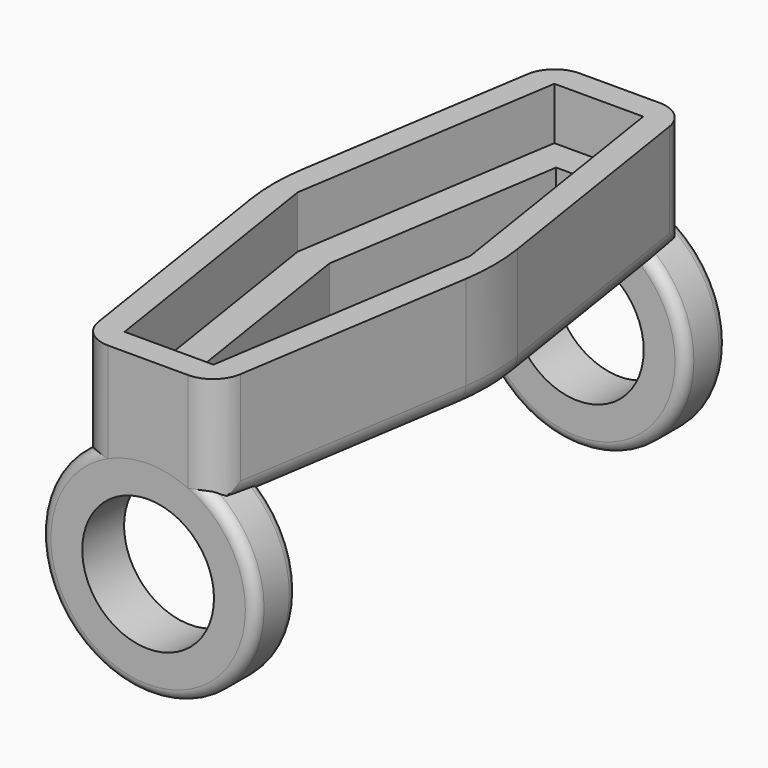
from build123d import *

# Parameters (mm, degrees)
F1_DEPTH     = 6
F2_DEPTH     = 11
F3_R         = 10.3
F4_DEPTH     = 5
F8_R         = 2
F9_R         = 1
F9_2_R       = 1
F10_T1_DEPTH = 21.8452325787
F11_T1_DEPTH = 18.7849894416
F11_T4_ANGLE = 17.6997661969
F11_T6_ANGLE = 17.6997661969


# Not quite as in the source:
# - a fillet or chamfer that OpenCascade refuses, or shapes differently, is made with other operations: its cross-section is extruded or revolved along the edge and cut away or added


with BuildPart() as f1:
    # F0 (on Top) → F1 (new body)
    with BuildSketch(Plane.XY):
        Polygon((4.25, -25.6904651573), (8.25, 0), (4.25, 25.6904651573), (0, 25.6904651573), (-4.25, 25.6904651573), (-8.25, 0), (-4.25, -25.6904651573), (0, -25.6904651573), align=None)
        Polygon((0, 22.6904651573), (1.6809534843, 22.6904651573), (5.2138541178, 0), (1.6809534843, -22.6904651573), (0, -22.6904651573), (-1.6809534843, -22.6904651573), (-5.2138541178, 0), (-1.6809534843, 22.6904651573), align=None, mode=Mode.SUBTRACT)
    extrude(amount=F1_DEPTH)

    # F0 (on Top) → F2 (join)
    with BuildSketch(Plane.XY):
        Polygon((-6.3908720964, 28.1904651573), (-10.7801215685, 0), (-6.3908720964, -28.1904651573), (0, -28.1904651573), (6.3908720964, -28.1904651573), (10.7801215685, 0), (6.3908720964, 28.1904651573), (0, 28.1904651573), align=None)
        Polygon((4.25, 25.6904651573), (8.25, 0), (4.25, -25.6904651573), (0, -25.6904651573), (-4.25, -25.6904651573), (-8.25, 0), (-4.25, 25.6904651573), (0, 25.6904651573), align=None, mode=Mode.SUBTRACT)
    extrude(amount=F2_DEPTH)

    # F8
    f8_edges = [f1.edges().sort_by_distance(p)[0] for p in [
        (-8.585497, -14.095233, 0),
        (-8.585497, 14.095233, 0),
        (8.585497, 14.095233, 0),
        (8.585497, -14.095233, 0),
    ]]
    fillet(f8_edges, radius=F8_R)

    # F10: fillet of radius 3 on 4 edges, made by hand

    # F10_s2 → F10_t1 (cut)
    with BuildSketch(Plane.XY.offset(-4.4226162893)):
        with BuildLine():
            ThreePointArc((-3.8218255807, -28.1904651573), (-5.7731564875, -27.4691287333), (-6.7861100219, -25.6520036189))
            Line((-6.7861100219, -25.6520036189), (-6.3908720964, -28.1904651573))
            Line((-6.3908720964, -28.1904651573), (-3.8218255807, -28.1904651573))
        make_face()
        with BuildLine():
            ThreePointArc((3.8218255807, -28.1904651573), (5.7731564875, -27.4691287333), (6.7861100219, -25.6520036189))
            Line((6.7861100219, -25.6520036189), (6.3908720964, -28.1904651573))
            Line((6.3908720964, -28.1904651573), (3.8218255807, -28.1904651573))
        make_face()
        with BuildLine():
            ThreePointArc((-3.8218255807, 28.1904651573), (-5.7731564875, 27.4691287333), (-6.7861100219, 25.6520036189))
            Line((-6.7861100219, 25.6520036189), (-6.3908720964, 28.1904651573))
            Line((-6.3908720964, 28.1904651573), (-3.8218255807, 28.1904651573))
        make_face()
        with BuildLine():
            ThreePointArc((3.8218255807, 28.1904651573), (5.7731564875, 27.4691287333), (6.7861100219, 25.6520036189))
            Line((6.7861100219, 25.6520036189), (6.3908720964, 28.1904651573))
            Line((6.3908720964, 28.1904651573), (3.8218255807, 28.1904651573))
        make_face()
    extrude(amount=F10_T1_DEPTH, mode=Mode.SUBTRACT)

    # F11: fillet of radius 20 on 2 edges, made by hand

    # F11_s2 → F11_t1 (cut)
    with BuildSketch(Plane.XY):
        with BuildLine():
            ThreePointArc((-10.3010452952, -3.0769230769), (-10.5391490203, 0), (-10.3010452952, 3.0769230769))
            Line((-10.3010452952, 3.0769230769), (-10.7801215685, 0))
            Line((-10.7801215685, 0), (-10.3010452952, -3.0769230769))
        make_face()
        with BuildLine():
            ThreePointArc((10.3010452952, 3.0769230769), (10.5391490203, 0), (10.3010452952, -3.0769230769))
            Line((10.3010452952, -3.0769230769), (10.7801215685, 0))
            Line((10.7801215685, 0), (10.3010452952, 3.0769230769))
        make_face()
    extrude(amount=F11_T1_DEPTH, mode=Mode.SUBTRACT)

    # F11_s3 → F11_t4 (revolve, cut)
    with BuildSketch(Plane(origin=(-0.223925467, 1.4381873518, 0), x_dir=(0, 0, 1), z_dir=(-0.1538461538, 0.9880948137, 0))):
        with BuildLine():
            ThreePointArc((0, 8.6517822134), (0.5857864376, 10.0659957758), (2, 10.6517822134))
            Line((2, 10.6517822134), (0, 10.6517822134))
            Line((0, 10.6517822134), (0, 8.6517822134))
        make_face()
    revolve(axis=Axis((-9.4608509797, 0, 0), (0, 0, -1)), revolution_arc=F11_T4_ANGLE, mode=Mode.SUBTRACT)

    # F11_s5 → F11_t6 (revolve, cut)
    with BuildSketch(Plane(origin=(0.223925467, -1.4381873518, 0), x_dir=(0, 0, 1), z_dir=(0.1538461538, -0.9880948137, 0))):
        with BuildLine():
            ThreePointArc((0, 8.6517822134), (0.5857864376, 10.0659957758), (2, 10.6517822134))
            Line((2, 10.6517822134), (0, 10.6517822134))
            Line((0, 10.6517822134), (0, 8.6517822134))
        make_face()
    revolve(axis=Axis((9.4608509797, 0, 0), (0, 0, -1)), revolution_arc=F11_T6_ANGLE, mode=Mode.SUBTRACT)


with BuildPart() as f4:
    # F3 (on face) → F4 (new body)
    with BuildSketch(Plane.XZ.offset(28.1904651573)):
        with Locations((0, -7)):
            Circle(F3_R)
        with BuildLine():
            ThreePointArc((0, -0.7), (4.4547727215, -2.5452272785), (6.3, -7))
            ThreePointArc((6.3, -7), (-4.4547727215, -11.4547727215), (0, -0.7))
        make_face(mode=Mode.SUBTRACT)
    extrude(amount=-F4_DEPTH)


with BuildPart() as f7_1:
    # F7: instance of F4
    add(f4.part.mirror(Plane(origin=(0, 0, -12.5), x_dir=(-1, 0, 0), z_dir=(0, -1, 0))))

    # F9#2
    f9_2_edges = [f7_1.edges().sort_by_distance(p)[0] for p in [
        (-10.3, 28.190465, -7),
        (-10.3, 23.190465, -7),
    ]]
    fillet(f9_2_edges, radius=F9_2_R)


with BuildPart() as f4_1:
    add(f4.part)

    # F9
    f9_edges = [f4_1.edges().sort_by_distance(p)[0] for p in [
        (-10.3, -28.190465, -7),
        (-10.3, -23.190465, -7),
    ]]
    fillet(f9_edges, radius=F9_R)


solid = Compound([f1.part, f7_1.part, f4_1.part])
